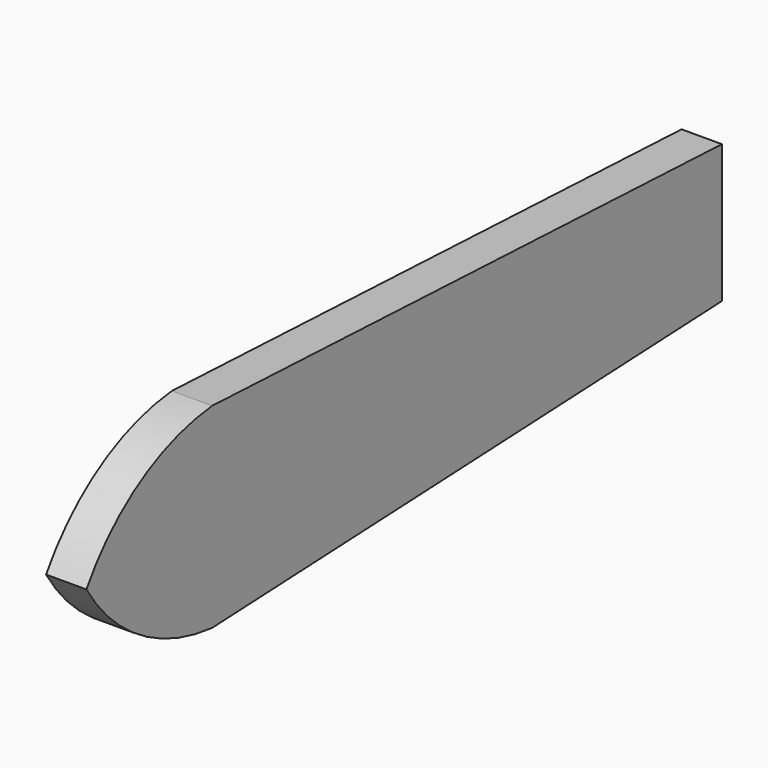
from build123d import *

# Parameters (mm, degrees)
F1_DEPTH = 6.858


# Not quite as in the source:
# - the program builds the solid bodies; features that only make, move or delete a surface that nothing else refers to are left out


with BuildPart() as f1:
    # F0 (on Right) → F1 (new body)
    with BuildSketch(Plane.YZ):
        with BuildLine():
            Line((61.0633231699, 11.7456540465), (-47.3298765719, 16.6299846023))
            ThreePointArc((-47.3298765719, 16.6299846023), (-62.6691287871, 11.4749888817), (-74.0792676806, 0))
            Line((-74.0792676806, 0), (61.0633231699, 0))
            Line((61.0633231699, 0), (61.0633231699, 11.7456540465))
        make_face()
        with BuildLine():
            Line((61.0633231699, 0), (-74.0792676806, 0))
            ThreePointArc((-74.0792676806, 0), (-62.6691287871, -11.4749888817), (-47.3298765719, -16.6299846023))
            Line((-47.3298765719, -16.6299846023), (61.0633231699, -11.7456540465))
            Line((61.0633231699, -11.7456540465), (61.0633231699, 0))
        make_face()
    extrude(amount=F1_DEPTH)


solid = f1.part
